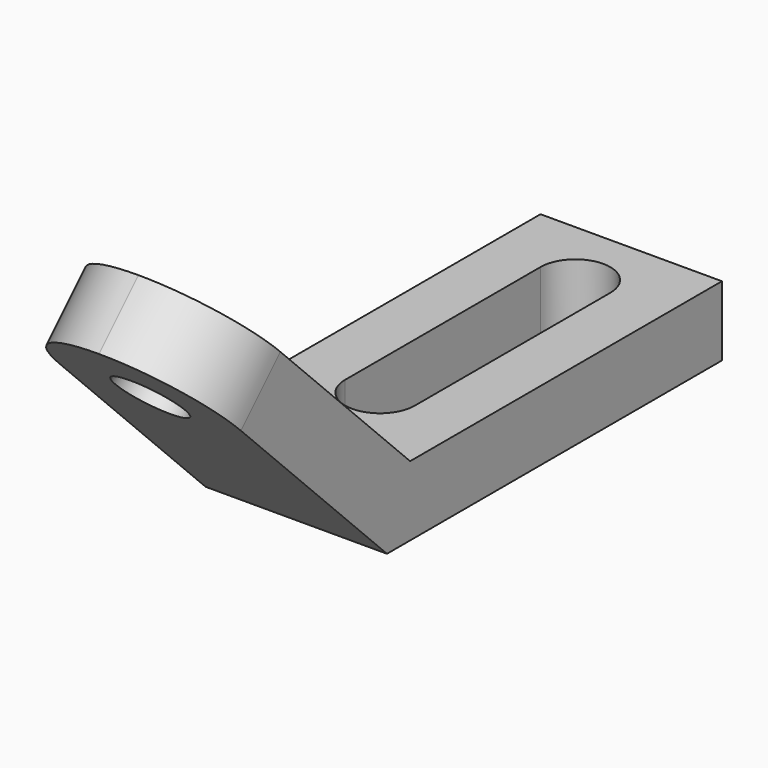
from build123d import *

# Parameters (mm, degrees)
F0_W     = 10
F0_H     = 20
F0_W_2   = 50
F2_DEPTH = 52
F3_R     = 25.99999
F4_D     = 20
F1_W     = 10
F1_H     = 70
F5_DEPTH = 47
F7_D     = 20


# Not quite as in the source:
# - a fillet or chamfer is up to 0.001 mm smaller than in the source, because OpenCascade refuses the exact size


with BuildPart() as f2:
    # F0 (on Right) → F2 (new body)
    with BuildSketch(Plane.YZ):
        with Locations((-5, 10)):
            Rectangle(F0_W, F0_H)
        with Locations((-15, 10)):
            Rectangle(F0_W, F0_H)
        with Locations((-25, 10)):
            Rectangle(F0_W, F0_H)
        with Locations((-55, 10)):
            Rectangle(F0_W_2, F0_H)
        with Locations((-85, 10)):
            Rectangle(F0_W, F0_H)
        with Locations((-95, 10)):
            Rectangle(F0_W, F0_H)
        Polygon((-120, 0), (-100, 0), (-100, 20), (-111.7157287525, 20), (-151.1126983722, 59.3969696197), (-165.2548339959, 45.2548339959), align=None)
        Polygon((-172.3259018078, 52.3259018078), (-165.2548339959, 45.2548339959), (-151.1126983722, 59.3969696197), (-158.1837661841, 66.4680374315), align=None)
        Polygon((-179.3969696197, 59.3969696197), (-172.3259018078, 52.3259018078), (-158.1837661841, 66.4680374315), (-165.2548339959, 73.5391052434), align=None)
        Polygon((-190.7106781187, 70.7106781187), (-179.3969696197, 59.3969696197), (-165.2548339959, 73.5391052434), (-176.5685424949, 84.8528137424), align=None)
    extrude(amount=F2_DEPTH)

    # F3 (radius 26 in the source; OpenCascade refuses exactly that, so slightly less here)
    f3_edges = [f2.edges().sort_by_distance(p)[0] for p in [
        (52, -183.63961, 77.781746),
        (0, -183.63961, 77.781746),
    ]]
    fillet(f3_edges, radius=F3_R)

    # F4 (through all)
    with Locations(Plane(origin=(0, 0, 0), x_dir=(1, 0, 0), z_dir=(0, 0, -1))):
        with Locations((26, 90.0006328523), (26, 20.0006328523)):
            Hole(F4_D / 2)

    # F1 (on Top) → F5 (cut)
    with BuildSketch(Plane.XY):
        with Locations((31, -55.0006328523)):
            Rectangle(F1_W, F1_H)
        with Locations((21, -55.0006328523)):
            Rectangle(F1_W, F1_H)
    extrude(amount=F5_DEPTH, mode=Mode.SUBTRACT)

    # F7 (through all)
    with Locations(Plane(origin=(0, -45.8578643763, -45.8578643763), x_dir=(-1, 0, 0), z_dir=(0, 0.7071067812, 0.7071067812))):
        with Locations((-26, 158.8528137424)):
            Hole(F7_D / 2)


solid = f2.part
